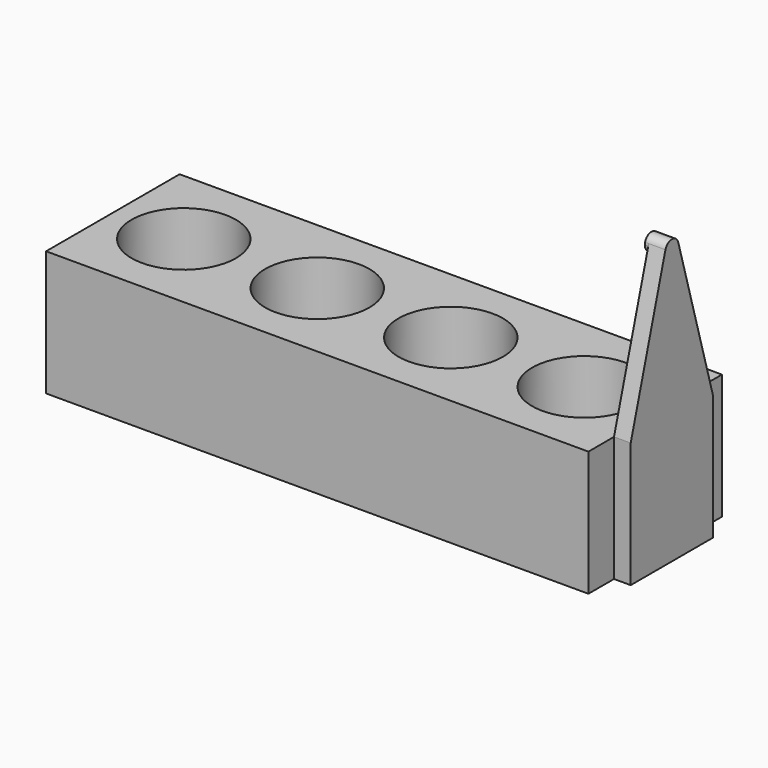
from build123d import *

# Parameters (mm, degrees)
F0_W     = 130
F0_H     = 40
F0_R     = 12.5
F1_DEPTH = 30
F2_W     = 12.3288280059
F2_H     = 30
F3_DEPTH = 4
F4_DEPTH = 4
F6_DEPTH = 0.88206


with BuildPart() as f1:
    # F0 (on Top) → F1 (new body)
    with BuildSketch(Plane.XY):
        Rectangle(F0_W, F0_H)
        with Locations((-48, 0)):
            Circle(F0_R, mode=Mode.SUBTRACT)
        with Locations((-16, 0)):
            Circle(F0_R, mode=Mode.SUBTRACT)
        with Locations((16, 0)):
            Circle(F0_R, mode=Mode.SUBTRACT)
        with Locations((48, 0)):
            Circle(F0_R, mode=Mode.SUBTRACT)
    extrude(amount=F1_DEPTH)

    # F2 (on face) → F3 (join)
    with BuildSketch(Plane.YZ.offset(65)):
        with BuildLine():
            Line((-12.3288280059, 30), (0, 30))
            Line((0, 30), (0, 64))
            ThreePointArc((0, 64), (-1.5961346024, 64.7948633558), (-1.9235602984, 66.5476456688))
            Line((-1.9235602984, 66.5476456688), (-12.3288280059, 30))
        make_face()
        with BuildLine():
            Line((0, 64), (0, 30))
            Line((0, 30), (12.3288280059, 30))
            Line((12.3288280059, 30), (1.9235602984, 66.5476456688))
            ThreePointArc((1.9235602984, 66.5476456688), (1.9807978944, 66.2764773076), (2, 66))
            ThreePointArc((2, 66), (1.4142135624, 64.5857864376), (0, 64))
        make_face()
        with Locations((6.164414003, 15)):
            Rectangle(F2_W, F2_H)
        with Locations((-6.164414003, 15)):
            Rectangle(F2_W, F2_H)
    extrude(amount=F3_DEPTH)

    # F2 (on face) → F4 (join)
    with BuildSketch(Plane.YZ.offset(65)):
        with BuildLine():
            Line((0, 0), (0, 30))
            Line((0, 30), (0, 64))
            ThreePointArc((0, 64), (-1.5961346024, 64.7948633558), (-1.9235602984, 66.5476456688))
            Line((-1.9235602984, 66.5476456688), (-12.3288280059, 30))
            Line((-12.3288280059, 30), (-12.3288280059, 0))
            Line((-12.3288280059, 0), (0, 0))
        make_face()
        with BuildLine():
            Line((0, 64), (0, 30))
            Line((0, 30), (0, 0))
            Line((0, 0), (12.3288280059, 0))
            Line((12.3288280059, 0), (12.3288280059, 30))
            Line((12.3288280059, 30), (1.9235602984, 66.5476456688))
            ThreePointArc((1.9235602984, 66.5476456688), (1.9807978944, 66.2764773076), (2, 66))
            ThreePointArc((2, 66), (1.4142135624, 64.5857864376), (0, 64))
        make_face()
        with BuildLine():
            ThreePointArc((-1.9235602984, 66.5476456688), (-1.5961346024, 64.7948633558), (0, 64))
            ThreePointArc((0, 64), (1.4142135624, 64.5857864376), (2, 66))
            ThreePointArc((2, 66), (1.9807978944, 66.2764773076), (1.9235602984, 66.5476456688))
            ThreePointArc((1.9235602984, 66.5476456688), (0, 68), (-1.9235602984, 66.5476456688))
        make_face()
    extrude(amount=F4_DEPTH)

    # F5 (on face) → F6 (join)
    with BuildSketch(Plane(origin=(65, 0, 0), x_dir=(0, -1, 0), z_dir=(-1, 0, 0))):
        with BuildLine():
            ThreePointArc((-1.9235602984, 66.5476456688), (-0.2764773076, 64.0192021056), (2, 66))
            ThreePointArc((2, 66), (1.9807978944, 66.2764773076), (1.9235602984, 66.5476456688))
            ThreePointArc((1.9235602984, 66.5476456688), (0, 68), (-1.9235602984, 66.5476456688))
        make_face()
    extrude(amount=F6_DEPTH)


solid = f1.part
